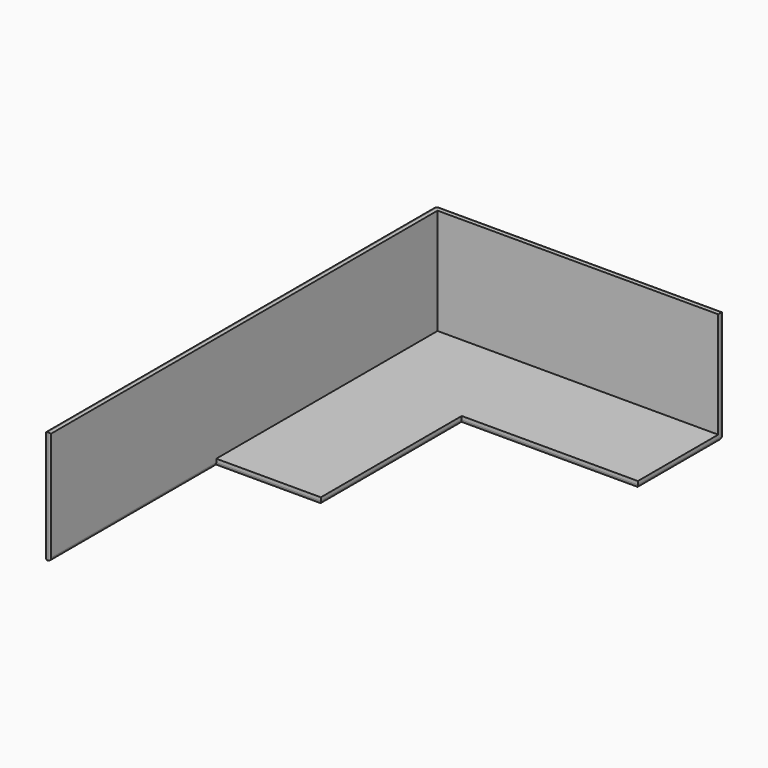
from build123d import *

# Parameters (mm, degrees)
F1_DEPTH     = 41
F3_DEPTH     = 38.5
F5_T1_DEPTH  = 38.46
F5_T3_DEPTH  = 179.905
F5_T5_DEPTH  = 106.405
F5_T7_DEPTH  = 47.35
F5_T9_DEPTH  = 42.905
F5_T11_DEPTH = 78.175
F5_T13_DEPTH = 41.175
F5_T15_DEPTH = 67.175
F5_T17_DEPTH = 67.175
F5_T19_DEPTH = 40.905
F5_T21_DEPTH = 101.96
F5_S25_W     = 1.27
F5_S25_H     = 1.27
F5_T26_DEPTH = 1.27
F5_S31_W     = 1.27
F5_S31_H     = 1.27
F5_T32_DEPTH = 1.27
F5_S37_W     = 1.27
F5_S37_H     = 1.27
F5_T38_DEPTH = 1.27
F5_T45_DEPTH = 81.35
F5_T49_DEPTH = 44.35
F5_T56_DEPTH = 70.35
F5_T60_DEPTH = 70.35


# Not quite as in the source:
# - a fillet or chamfer that OpenCascade refuses, or shapes differently, is made with other operations: its cross-section is extruded or revolved along the edge and cut away or added
# - a feature of the source that left no trace in its solid (it failed there, or was rolled back) is left out


with BuildPart() as f1:
    # F0 (on Top) → F1 (new body)
    with BuildSketch(Plane.XY):
        Polygon((0, 102.9857128358), (0, 0), (0, -75.0142871642), (2.5, -75.0142871642), (2.5, -0.0142871642), (40.5, -0.0142871642), (40.5, 63.9857128358), (104.5, 63.9857128358), (104.5, 102.9857128358), align=None)
    extrude(amount=F1_DEPTH)

    # F2 (on face) → F3 (cut)
    with BuildSketch(Plane.XY.offset(41)):
        Polygon((2.5, 100.4857128358), (2.5, -0.0142871642), (40.5, -0.0142871642), (40.5, 63.9857128358), (104.5, 63.9857128358), (104.5, 100.4857128358), align=None)
    extrude(amount=-F3_DEPTH, mode=Mode.SUBTRACT)

    # F5: fillet of radius 1.27 on 12 edges, made by hand

    # F5_s2 → F5_t1 (cut)
    with BuildSketch(Plane.XY.offset(1.27)):
        with BuildLine():
            ThreePointArc((0, 101.7157128358), (0.3719743879, 102.6137384479), (1.27, 102.9857128358))
            Line((1.27, 102.9857128358), (0, 102.9857128358))
            Line((0, 102.9857128358), (0, 101.7157128358))
        make_face()
    extrude(amount=F5_T1_DEPTH, mode=Mode.SUBTRACT)

    # F5_s4 → F5_t3 (cut)
    with BuildSketch(Plane.XZ.offset(-101.7157128358)):
        with BuildLine():
            ThreePointArc((0, 39.73), (0.3719743879, 40.6280256121), (1.27, 41))
            Line((1.27, 41), (0, 41))
            Line((0, 41), (0, 39.73))
        make_face()
        with BuildLine():
            ThreePointArc((0, 1.27), (0.3719743879, 0.3719743879), (1.27, 0))
            Line((1.27, 0), (0, 0))
            Line((0, 0), (0, 1.27))
        make_face()
    extrude(amount=F5_T3_DEPTH, mode=Mode.SUBTRACT)

    # F5_s6 → F5_t5 (cut)
    with BuildSketch(Plane.YZ.offset(1.27)):
        with BuildLine():
            ThreePointArc((101.7157128358, 41), (102.6137384479, 40.6280256121), (102.9857128358, 39.73))
            Line((102.9857128358, 39.73), (102.9857128358, 41))
            Line((102.9857128358, 41), (101.7157128358, 41))
        make_face()
    extrude(amount=F5_T5_DEPTH, mode=Mode.SUBTRACT)

    # F5_s8 → F5_t7 (cut)
    with BuildSketch(Plane.XY.offset(-3.175)):
        with BuildLine():
            ThreePointArc((0, -73.7442871642), (0.3719743879, -74.6423127763), (1.27, -75.0142871642))
            Line((1.27, -75.0142871642), (0, -75.0142871642))
            Line((0, -75.0142871642), (0, -73.7442871642))
        make_face()
    extrude(amount=F5_T7_DEPTH, mode=Mode.SUBTRACT)

    # F5_s10 → F5_t9 (cut)
    with BuildSketch(Plane.XY.offset(1.27)):
        with BuildLine():
            ThreePointArc((104.5, 101.7157128358), (104.1280256121, 102.6137384479), (103.23, 102.9857128358))
            Line((103.23, 102.9857128358), (104.5, 102.9857128358))
            Line((104.5, 102.9857128358), (104.5, 101.7157128358))
        make_face()
    extrude(amount=F5_T9_DEPTH, mode=Mode.SUBTRACT)

    # F5_s12 → F5_t11 (cut)
    with BuildSketch(Plane.XZ.offset(0.0142871642)):
        with BuildLine():
            ThreePointArc((1.23, 0), (2.1280256121, 0.3719743879), (2.5, 1.27))
            Line((2.5, 1.27), (2.5, 0))
            Line((2.5, 0), (1.23, 0))
        make_face()
    extrude(amount=F5_T11_DEPTH, mode=Mode.SUBTRACT)

    # F5_s14 → F5_t13 (cut)
    with BuildSketch(Plane.YZ.offset(2.5)):
        with BuildLine():
            ThreePointArc((1.2557128358, 0), (0.3576872237, 0.3719743879), (-0.0142871642, 1.27))
            Line((-0.0142871642, 1.27), (-0.0142871642, 0))
            Line((-0.0142871642, 0), (1.2557128358, 0))
        make_face()
    extrude(amount=F5_T13_DEPTH, mode=Mode.SUBTRACT)

    # F5_s16 → F5_t15 (cut)
    with BuildSketch(Plane.XZ.offset(-63.9857128358)):
        with BuildLine():
            ThreePointArc((39.23, 0), (40.1280256121, 0.3719743879), (40.5, 1.27))
            Line((40.5, 1.27), (40.5, 0))
            Line((40.5, 0), (39.23, 0))
        make_face()
    extrude(amount=F5_T15_DEPTH, mode=Mode.SUBTRACT)

    # F5_s18 → F5_t17 (cut)
    with BuildSketch(Plane.YZ.offset(40.5)):
        with BuildLine():
            ThreePointArc((65.2557128358, 0), (64.3576872237, 0.3719743879), (63.9857128358, 1.27))
            Line((63.9857128358, 1.27), (63.9857128358, 0))
            Line((63.9857128358, 0), (65.2557128358, 0))
        make_face()
    extrude(amount=F5_T17_DEPTH, mode=Mode.SUBTRACT)

    # F5_s20 → F5_t19 (cut)
    with BuildSketch(Plane.XZ.offset(-101.7157128358)):
        with BuildLine():
            ThreePointArc((103.23, 0), (104.1280256121, 0.3719743879), (104.5, 1.27))
            Line((104.5, 1.27), (104.5, 0))
            Line((104.5, 0), (103.23, 0))
        make_face()
    extrude(amount=F5_T19_DEPTH, mode=Mode.SUBTRACT)

    # F5_s22 → F5_t21 (cut)
    with BuildSketch(Plane.YZ.offset(1.27)):
        with BuildLine():
            ThreePointArc((101.7157128358, 0), (102.6137384479, 0.3719743879), (102.9857128358, 1.27))
            Line((102.9857128358, 1.27), (102.9857128358, 0))
            Line((102.9857128358, 0), (101.7157128358, 0))
        make_face()
    extrude(amount=F5_T21_DEPTH, mode=Mode.SUBTRACT)


with BuildPart() as f5_tool24:
    # F5_s25 → F5_t26 (new body)
    with BuildSketch(Plane.YZ.offset(1.27)):
        with Locations((102.3507128358, 0.635)):
            Rectangle(F5_S25_W, F5_S25_H)
    extrude(amount=-F5_T26_DEPTH)

    # F5_s27 → F5_t28 (revolve, cut)
    with BuildSketch(Plane(origin=(1.27, 101.7157128358, 1.27), x_dir=(0, -0.7071067812, 0.7071067812), z_dir=(0, -0.7071067812, -0.7071067812))):
        with BuildLine():
            ThreePointArc((0, -1.27), (1.27, 0), (0, 1.27))
            Line((0, 1.27), (0, -1.27))
        make_face()
    revolve(axis=Axis((1.27, 101.7157128358, 1.27), (-1, 0, 0)), mode=Mode.SUBTRACT)


with BuildPart() as f1_1:
    add(f1.part)

    # F5_t23: cut F5_tool24
    add(f5_tool24.part, mode=Mode.SUBTRACT)


with BuildPart() as f5_tool30:
    # F5_s31 → F5_t32 (new body)
    with BuildSketch(Plane.YZ.offset(1.27)):
        with Locations((102.3507128358, 40.365)):
            Rectangle(F5_S31_W, F5_S31_H)
    extrude(amount=-F5_T32_DEPTH)

    # F5_s33 → F5_t34 (revolve, cut)
    with BuildSketch(Plane(origin=(1.27, 101.7157128358, 39.73), x_dir=(0, -0.7071067812, -0.7071067812), z_dir=(0, 0.7071067812, -0.7071067812))):
        with BuildLine():
            ThreePointArc((0, -1.27), (1.27, 0), (0, 1.27))
            Line((0, 1.27), (0, -1.27))
        make_face()
    revolve(axis=Axis((1.27, 101.7157128358, 39.73), (-1, 0, 0)), mode=Mode.SUBTRACT)


with BuildPart() as f1_2:
    add(f1_1.part)

    # F5_t29: cut F5_tool30
    add(f5_tool30.part, mode=Mode.SUBTRACT)


with BuildPart() as f5_tool36:
    # F5_s37 → F5_t38 (new body)
    with BuildSketch(Plane.XY.offset(1.27)):
        with Locations((103.865, 102.3507128358)):
            Rectangle(F5_S37_W, F5_S37_H)
    extrude(amount=-F5_T38_DEPTH)

    # F5_s39 → F5_t40 (revolve, cut)
    with BuildSketch(Plane(origin=(103.23, 101.7157128358, 1.27), x_dir=(-0.7071067812, -0.7071067812, 0), z_dir=(0.7071067812, -0.7071067812, 0))):
        with BuildLine():
            ThreePointArc((0, -1.27), (1.27, 0), (0, 1.27))
            Line((0, 1.27), (0, -1.27))
        make_face()
    revolve(axis=Axis((103.23, 101.7157128358, 1.27), (0, 0, -1)), mode=Mode.SUBTRACT)


with BuildPart() as f1_3:
    add(f1_2.part)

    # F5_t35: cut F5_tool36
    add(f5_tool36.part, mode=Mode.SUBTRACT)


with BuildPart() as f5_tool43:
    # F5_s44 → F5_t45 (new body)
    with BuildSketch(Plane.XZ.offset(78.1892871642)):
        with BuildLine():
            ThreePointArc((1.23, 0), (2.1280256121, 0.3719743879), (2.5, 1.27))
            Line((2.5, 1.27), (2.5, 0))
            Line((2.5, 0), (1.23, 0))
        make_face()
    extrude(amount=-F5_T45_DEPTH)

    split(bisect_by=Plane.XZ.offset(0.0142871642), keep=Keep.BOTTOM)


with BuildPart() as f5_tool47:
    # F5_s48 → F5_t49 (new body)
    with BuildSketch(Plane.YZ.offset(-0.675)):
        with BuildLine():
            ThreePointArc((1.2557128358, 0), (0.3576872237, 0.3719743879), (-0.0142871642, 1.27))
            Line((-0.0142871642, 1.27), (-0.0142871642, 0))
            Line((-0.0142871642, 0), (1.2557128358, 0))
        make_face()
    extrude(amount=F5_T49_DEPTH)

    split(bisect_by=Plane.YZ.offset(2.5), keep=Keep.BOTTOM)


with BuildPart() as f5_tool43_1:
    add(f5_tool43.part)

    # F5_t51: intersect F5_tool47
    add(f5_tool47.part, mode=Mode.INTERSECT)


with BuildPart() as f1_4:
    add(f1_3.part)

    # F5_t41: cut F5_tool43
    add(f5_tool43_1.part, mode=Mode.SUBTRACT)


with BuildPart() as f5_tool54:
    # F5_s55 → F5_t56 (new body)
    with BuildSketch(Plane.XZ.offset(3.1892871642)):
        with BuildLine():
            ThreePointArc((39.23, 0), (40.1280256121, 0.3719743879), (40.5, 1.27))
            Line((40.5, 1.27), (40.5, 0))
            Line((40.5, 0), (39.23, 0))
        make_face()
    extrude(amount=-F5_T56_DEPTH)

    split(bisect_by=Plane.XZ.offset(-63.9857128358), keep=Keep.BOTTOM)


with BuildPart() as f5_tool58:
    # F5_s59 → F5_t60 (new body)
    with BuildSketch(Plane.YZ.offset(37.325)):
        with BuildLine():
            ThreePointArc((65.2557128358, 0), (64.3576872237, 0.3719743879), (63.9857128358, 1.27))
            Line((63.9857128358, 1.27), (63.9857128358, 0))
            Line((63.9857128358, 0), (65.2557128358, 0))
        make_face()
    extrude(amount=F5_T60_DEPTH)

    split(bisect_by=Plane.YZ.offset(40.5), keep=Keep.BOTTOM)


with BuildPart() as f5_tool54_1:
    add(f5_tool54.part)

    # F5_t62: intersect F5_tool58
    add(f5_tool58.part, mode=Mode.INTERSECT)


with BuildPart() as f1_5:
    add(f1_4.part)

    # F5_t52: cut F5_tool54
    add(f5_tool54_1.part, mode=Mode.SUBTRACT)


solid = f1_5.part
